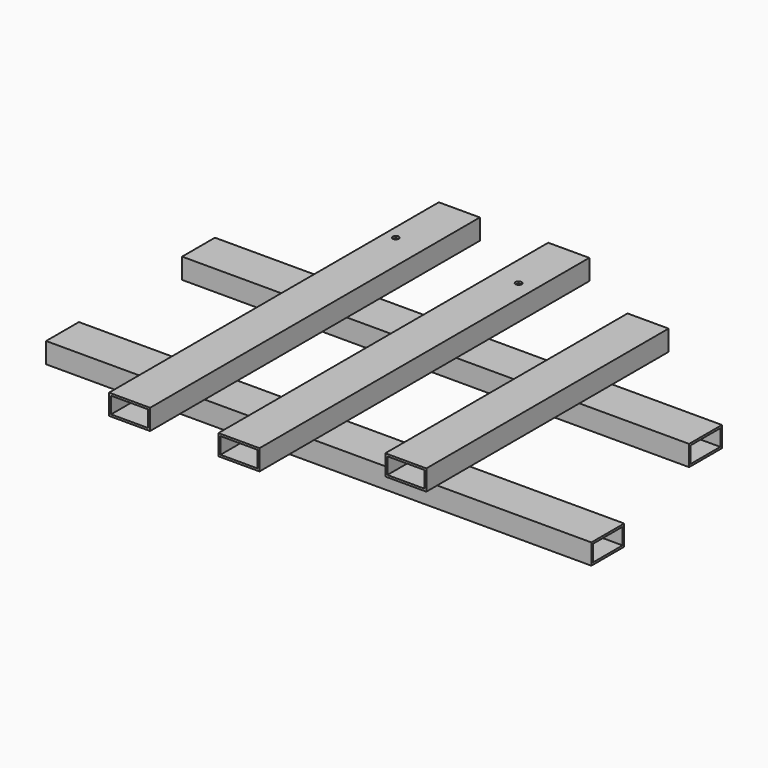
from build123d import *

# Parameters (mm, degrees)
F0_W        = 60
F0_H        = 30
F1_DEPTH    = 158
F2_W        = 66.2892647088
F2_H        = 29.4618904591
F3_DEPTH    = 300
F2_W_2      = 68.393683061
F2_H_2      = 30.5141024292
F2_W_3      = 67.3414766788
F4_W        = 47.0454245806
F4_H        = 22.7635130286
F5_DEPTH    = 400
F4_W_2      = 49.3977004662
F4_H_2      = 23.8089710474
F6_DEPTH    = 50
F7_W        = 61.1065607518
F7_H        = 23.5696807504
F8_DEPTH    = 300
F9_W        = 60.6583654881
F9_H        = 23.7780623138
F9_W_2      = 61.8215240538
F9_H_2      = 23.7314254045
F10_DEPTH   = 300.001
F11_W       = 61.2598918378
F11_H       = 23.6744321883
F12_DEPTH   = 300.001
F13_W       = 41.8233666569
F13_H       = 17.940826714
F14_DEPTH   = 450.001
F15_W       = 0.6950423121
F15_H       = 16.4160877466
F15_W_2     = 41.8233666569
F15_W_3     = 0.0805514865
F16_DEPTH   = 450.001
F18_R       = 8.0737977812
F18_R_2     = 2.2693206324
F19_DEPTH   = 10
F21_W       = 60
F21_H       = 177.2603205867
F21_H_2     = 60
F21_H_3     = 180
F21_H_4     = 125.5965695061
F22_DEPTH   = 30
F21_H_5     = 97.260340693
F21_H_6     = 45.5965896123
F23_W       = 797.4684381369
F23_H       = 60
F24_DEPTH   = 30
F23_W_2     = 826.1469494374
F25_W       = 54.0000002086
F25_H       = 24.0000002086
F26_DEPTH   = 877.8865025663
F27_W       = 54.0000002086
F27_H       = 24.0000002086
F28_DEPTH   = 868.8368023466
F29_W       = 54.000005275
F29_H       = 24.000005275
F30_DEPTH   = 602.8578900928
F31_W       = 54.000005275
F31_H       = 24.000005275
F32_DEPTH   = 602.8578900928
F33_W       = 54.000005275
F33_H       = 24.000005275
F34_DEPTH   = 522.857910199
F35_DEPTH   = 153.3
F37_DEPTH   = 68.6
F40_D       = 8.8
F40_DEPTH   = 16.5
F40_TIP     = 2.6437867237
F40_2_D     = 8.8
F40_2_DEPTH = 16.5
F40_2_TIP   = 2.6437867237
F41_D       = 8.8
F41_DEPTH   = 16.5
F41_TIP     = 2.6437867237
F41_2_D     = 8.8
F41_2_DEPTH = 16.5
F41_2_TIP   = 2.6437867237


# Not quite as in the source:
# - a feature names something its author has since deleted; it is built from what else it names


with BuildPart() as f1:
    # F0 (on Right) → F1 (new body)
    with BuildSketch(Plane.YZ):
        with Locations((-26.7016614429, 57.4951861054)):
            Rectangle(F0_W, F0_H)
    extrude(amount=F1_DEPTH)


with BuildPart() as f3:
    # F2 (on face) → F3 (new body)
    with BuildSketch(Plane.XZ.offset(56.7016614429)):
        with Locations((-55.3080569953, -72.8603079915)):
            Rectangle(F2_W, F2_H)
    extrude(amount=-F3_DEPTH)

    # F7 (on face) → F8 (cut, through all)
    with BuildSketch(Plane.XZ.offset(56.7016614429)):
        with Locations((-55.1617154852, -72.5816227496)):
            Rectangle(F7_W, F7_H)
    extrude(amount=-F8_DEPTH, mode=Mode.SUBTRACT)


with BuildPart() as f3b:
    # F2 (on face) → F3, piece 2 (new body)
    with BuildSketch(Plane.XZ.offset(56.7016614429)):
        with Locations((56.2262581661, -72.3342020065)):
            Rectangle(F2_W_2, F2_H_2)
    extrude(amount=-F3_DEPTH)


with BuildPart() as f3c:
    # F2 (on face) → F3, piece 3 (new body)
    with BuildSketch(Plane.XZ.offset(56.7016614429)):
        with Locations((181.9654107094, -72.3342020065)):
            Rectangle(F2_W_3, F2_H_2)
    extrude(amount=-F3_DEPTH)


with BuildPart() as f5:
    # F4 (on face) → F5 (new body)
    with BuildSketch(Plane(origin=(-88.4526893497, 0, 0), x_dir=(0, -1, 0), z_dir=(-1, 0, 0))):
        with Locations((-189.4800886512, -98.9730097353)):
            Rectangle(F4_W, F4_H)
    extrude(amount=-F5_DEPTH)


with BuildPart() as f5b:
    # F4 (on face) → F5, piece 2 (new body)
    with BuildSketch(Plane(origin=(-88.4526893497, 0, 0), x_dir=(0, -1, 0), z_dir=(-1, 0, 0))):
        with Locations((-13.9745208435, -99.4957387447)):
            Rectangle(F4_W_2, F4_H_2)
    extrude(amount=-F5_DEPTH)


with BuildPart() as f6:
    # F6 (new): a face of the model
    f6_faces = [f5.part.faces().sort_by_distance(p)[0] for p in [
        (-88.4526893497, 189.4800886512, -98.9730097353),
    ]]
    extrude(f6_faces, amount=F6_DEPTH)


with BuildPart() as f6b:
    # F6#2 (new): a face of the model
    f6_2_faces = [f5b.part.faces().sort_by_distance(p)[0] for p in [
        (-88.4526893497, 13.9745208435, -99.4957387447),
    ]]
    extrude(f6_2_faces, amount=F6_DEPTH)


with BuildPart() as f10_tool:
    # F9 (on face) → F10 (new body, through all)
    with BuildSketch(Plane.XZ.offset(56.7016614429)):
        with Locations((181.9215863943, -72.4789816886)):
            Rectangle(F9_W, F9_H)
        with Locations((56.3811119646, -72.2706690431)):
            Rectangle(F9_W_2, F9_H_2)
    extrude(amount=-F10_DEPTH)


with BuildPart() as f3b_1:
    add(f3b.part)

    # F10: cut by f10_tool
    add(f10_tool.part, mode=Mode.SUBTRACT)

    # F11 (on face) → F12 (cut, through all)
    with BuildSketch(Plane.XZ.offset(56.7016614429)):
        with Locations((55.9759307653, -72.5225340575)):
            Rectangle(F11_W, F11_H)
    extrude(amount=-F12_DEPTH, mode=Mode.SUBTRACT)


with BuildPart() as f3c_1:
    add(f3c.part)

    # F10: cut by f10_tool
    add(f10_tool.part, mode=Mode.SUBTRACT)


with BuildPart() as f14_tool:
    # F13 (on face) → F14 (new body, through all)
    with BuildSketch(Plane.YZ.offset(311.5473106503)):
        with Locations((13.9583600685, -99.7032783926)):
            Rectangle(F13_W, F13_H)
    extrude(amount=-F14_DEPTH)


with BuildPart() as f5b_1:
    add(f5b.part)

    # F14: cut by f14_tool
    add(f14_tool.part, mode=Mode.SUBTRACT)


with BuildPart() as f6b_1:
    add(f6b.part)

    # F14: cut by f14_tool
    add(f14_tool.part, mode=Mode.SUBTRACT)


with BuildPart() as f16_tool:
    # F15 (on face) → F16 (new body, through all)
    with BuildSketch(Plane(origin=(-138.4526893497, 0, 0), x_dir=(0, -1, 0), z_dir=(-1, 0, 0))):
        with Locations((-35.217564553, -99.4463041425)):
            Rectangle(F15_W, F15_H)
        with Locations((-13.9583600685, -99.4463041425)):
            Rectangle(F15_W_2, F15_H)
        with Locations((6.9935990032, -99.4463041425)):
            Rectangle(F15_W_3, F15_H)
    extrude(amount=-F16_DEPTH)


with BuildPart() as f5b_2:
    add(f5b_1.part)

    # F16: cut by f16_tool
    add(f16_tool.part, mode=Mode.SUBTRACT)


with BuildPart() as f6b_2:
    add(f6b_1.part)

    # F16: cut by f16_tool
    add(f16_tool.part, mode=Mode.SUBTRACT)


with BuildPart() as f19:
    # F18 (on face) → F19 (new body)
    with BuildSketch(Plane.XY.offset(72.4951861054)):
        with Locations((62.8524050117, -9.2268595472)):
            Circle(F18_R)
        with Locations((59.0920038521, -6.9042602554)):
            Circle(F18_R_2, mode=Mode.SUBTRACT)
    extrude(amount=F19_DEPTH)


with BuildPart() as f22:
    # F21 (on face) → F22 (new body)
    with BuildSketch(Plane.XY.offset(72.4951861054)):
        with Locations((-508.9146799214, 155.734451874)):
            Rectangle(F21_W, F21_H)
        with Locations((-508.9146799214, 37.1042915806)):
            Rectangle(F21_W, F21_H_2)
        with Locations((-508.9146799214, -82.8957084194)):
            Rectangle(F21_W, F21_H_3)
        with Locations((-508.9146799214, -202.8957084194)):
            Rectangle(F21_W, F21_H_2)
        with Locations((-508.9146799214, -295.6939931724)):
            Rectangle(F21_W, F21_H_4)
    extrude(amount=F22_DEPTH)

    # F29 (on face) → F30 (cut, through all)
    with BuildSketch(Plane.XZ.offset(358.4922779254)):
        with Locations((-508.9146799214, 87.4951861054)):
            Rectangle(F29_W, F29_H)
    extrude(amount=-F30_DEPTH, mode=Mode.SUBTRACT)

    # F40
    with Locations(Plane.XY.offset(102.4951861054)):
        with Locations((-522.6472080988, 145.1861311495), (-342.6472080988, 145.1861311495)):
            Hole(F40_D / 2, depth=F40_DEPTH)
            with Locations((0, 0, -(F40_DEPTH + F40_TIP / 2))):  # 118° drill point
                Cone(0, F40_D / 2, F40_TIP, mode=Mode.SUBTRACT)

    # F41
    with Locations(Plane.XY.offset(102.4951861054)):
        with Locations((-522.6888656616, 145.43607831), (-342.8764343262, 145.0610905886)):
            Hole(F41_D / 2, depth=F41_DEPTH)
            with Locations((0, 0, -(F41_DEPTH + F41_TIP / 2))):  # 118° drill point
                Cone(0, F41_D / 2, F41_TIP, mode=Mode.SUBTRACT)


with BuildPart() as f22b:
    # F21 (on face) → F22, piece 2 (new body)
    with BuildSketch(Plane.XY.offset(72.4951861054)):
        with Locations((-348.9146799214, -295.6939931724)):
            Rectangle(F21_W, F21_H_4)
        with Locations((-348.9146799214, -202.8957084194)):
            Rectangle(F21_W, F21_H_2)
        with Locations((-348.9146799214, -82.8957084194)):
            Rectangle(F21_W, F21_H_3)
        with Locations((-348.9146799214, 37.1042915806)):
            Rectangle(F21_W, F21_H_2)
        with Locations((-348.9146799214, 155.734451874)):
            Rectangle(F21_W, F21_H)
    extrude(amount=F22_DEPTH)

    # F31 (on face) → F32 (cut, through all)
    with BuildSketch(Plane.XZ.offset(358.4922779254)):
        with Locations((-348.9146799214, 87.4951861054)):
            Rectangle(F31_W, F31_H)
    extrude(amount=-F32_DEPTH, mode=Mode.SUBTRACT)

    # F40#2
    with Locations(Plane.XY.offset(102.4951861054)):
        with Locations((-522.6472080988, 145.1861311495), (-342.6472080988, 145.1861311495)):
            Hole(F40_2_D / 2, depth=F40_2_DEPTH)
            with Locations((0, 0, -(F40_2_DEPTH + F40_2_TIP / 2))):  # 118° drill point
                Cone(0, F40_2_D / 2, F40_2_TIP, mode=Mode.SUBTRACT)

    # F41#2
    with Locations(Plane.XY.offset(102.4951861054)):
        with Locations((-522.6888656616, 145.43607831), (-342.8764343262, 145.0610905886)):
            Hole(F41_2_D / 2, depth=F41_2_DEPTH)
            with Locations((0, 0, -(F41_2_DEPTH + F41_2_TIP / 2))):  # 118° drill point
                Cone(0, F41_2_D / 2, F41_2_TIP, mode=Mode.SUBTRACT)


with BuildPart() as f22c:
    # F21 (on face) → F22, piece 3 (new body)
    with BuildSketch(Plane.XY.offset(72.4951861054)):
        with Locations((-168.9146799214, 115.7344619271)):
            Rectangle(F21_W, F21_H_5)
        with Locations((-168.9146799214, 37.1042915806)):
            Rectangle(F21_W, F21_H_2)
        with Locations((-168.9146799214, -82.8957084194)):
            Rectangle(F21_W, F21_H_3)
        with Locations((-168.9146799214, -202.8957084194)):
            Rectangle(F21_W, F21_H_2)
        with Locations((-168.9146799214, -255.6940032255)):
            Rectangle(F21_W, F21_H_6)
    extrude(amount=F22_DEPTH)

    # F33 (on face) → F34 (cut, through all)
    with BuildSketch(Plane.XZ.offset(278.4922980317)):
        with Locations((-168.9146799214, 87.4951861054)):
            Rectangle(F33_W, F33_H)
    extrude(amount=-F34_DEPTH, mode=Mode.SUBTRACT)


with BuildPart() as f24:
    # F23 (on face) → F24 (new body)
    with BuildSketch(Plane(origin=(0, 0, 72.4951861054), x_dir=(1, 0, 0), z_dir=(0, 0, -1))):
        with Locations((-312.1015832781, 228.705952694)):
            Rectangle(F23_W, F23_H)
    extrude(amount=F24_DEPTH)

    # F27 (on face) → F28 (cut, through all)
    with BuildSketch(Plane(origin=(-710.8358023466, 0, 0), x_dir=(0, -1, 0), z_dir=(-1, 0, 0))):
        with Locations((228.705952694, 57.4951861054)):
            Rectangle(F27_W, F27_H)
    extrude(amount=-F28_DEPTH, mode=Mode.SUBTRACT)


with BuildPart() as f24b:
    # F23 (on face) → F24, piece 2 (new body)
    with BuildSketch(Plane(origin=(0, 0, 72.4951861054), x_dir=(1, 0, 0), z_dir=(0, 0, -1))):
        with Locations((-306.8120278476, -31.294047306)):
            Rectangle(F23_W_2, F23_H)
    extrude(amount=F24_DEPTH)

    # F25 (on face) → F26 (cut, through all)
    with BuildSketch(Plane(origin=(-719.8855025663, 0, 0), x_dir=(0, -1, 0), z_dir=(-1, 0, 0))):
        with Locations((-31.294047306, 57.4951861054)):
            Rectangle(F25_W, F25_H)
    extrude(amount=-F26_DEPTH, mode=Mode.SUBTRACT)


with BuildPart() as f35_tool:
    # F35 (cut): a face of the model
    f35_faces = [f24b.part.faces().sort_by_distance(p)[0] for p in [
        (106.2614468711, 60.6232269128, 57.4951861054),
    ]]
    extrude(f35_faces, amount=-F35_DEPTH)


with BuildPart() as f1_1:
    add(f1.part)

    # F35: cut by f35_tool
    add(f35_tool.part, mode=Mode.SUBTRACT)


with BuildPart() as f24b_1:
    add(f24b.part)

    # F35: cut by f35_tool
    add(f35_tool.part, mode=Mode.SUBTRACT)

    # F37 (add): a face of the model
    f37_faces = [f24b_1.faces().sort_by_distance(p)[0] for p in [
        (-47.0385531289, 60.6232269128, 57.4951861054),
    ]]
    extrude(f37_faces, amount=F37_DEPTH)


solid = Compound([f22.part, f22b.part, f22c.part, f24.part, f24b_1.part])
